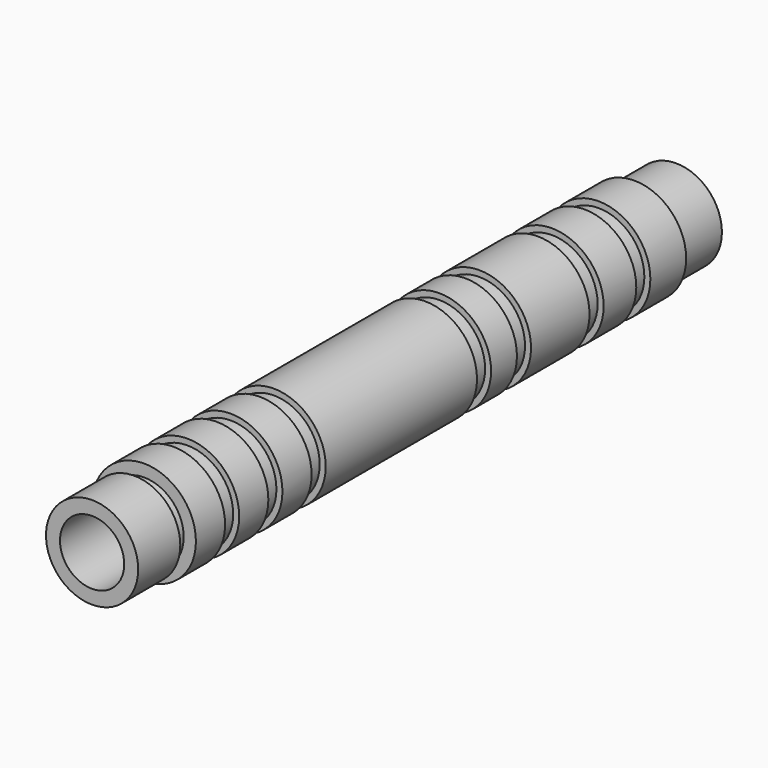
from build123d import *

# Parameters (mm, degrees)
F0_R         = 6.35
F1_DEPTH     = 46.9138
F2_R         = 3.048
F3_DEPTH     = 71.12
F4_R         = 3.937
F5_DEPTH     = 12.3698
F6_R         = 6.35
F6_R_2       = 5.6515
F7_DEPTH     = 6.4516
F8_R         = 6.35
F8_R_2       = 4.8514
F9_DEPTH     = 1.524
F10_S5_R     = 3.937
F10_T6_DEPTH = 7
F12_R        = 6.35
F12_R_2      = 5.6134
F13_DEPTH    = 2.159
F15_R        = 6.35
F15_R_2      = 5.6134
F16_DEPTH    = 2.159
F18_R        = 6.35
F18_R_2      = 5.6134
F19_DEPTH    = 2.159
F21_R        = 6.35
F21_R_2      = 5.6134
F22_DEPTH    = 2.159
F24_R        = 6.35
F24_R_2      = 5.6134
F25_DEPTH    = 2.159
F27_R        = 6.35
F27_R_2      = 5.6134
F28_DEPTH    = 2.159
F30_R        = 6.35
F30_R_2      = 5.6134
F31_DEPTH    = 2.159
F33_R        = 6.35
F33_R_2      = 5.6134
F34_DEPTH    = 10.7198
F35_SIZE2    = 5.6134
F35_SIZE     = 4.318


# Not quite as in the source:
# - a fillet or chamfer that OpenCascade refuses, or shapes differently, is made with other operations: its cross-section is extruded or revolved along the edge and cut away or added


with BuildPart() as f1:
    # F0 (on Front) → F1 (new body, symmetric)
    with BuildSketch(Plane.XZ):
        Circle(F0_R)
    extrude(amount=F1_DEPTH, both=True)

    # F2 (on face) → F3 (cut)
    with BuildSketch(Plane.XZ.offset(46.9138)):
        Circle(F2_R)
    extrude(amount=-F3_DEPTH, mode=Mode.SUBTRACT)

    # F4 (on face) → F5 (cut)
    with BuildSketch(Plane.XZ.offset(46.9138)):
        Circle(F4_R)
    extrude(amount=-F5_DEPTH, mode=Mode.SUBTRACT)

    # F6 (on face) → F7 (cut)
    with BuildSketch(Plane.XZ.offset(46.9138)):
        Circle(F6_R)
        Circle(F6_R_2, mode=Mode.SUBTRACT)
    extrude(amount=-F7_DEPTH, mode=Mode.SUBTRACT)

    # F8 (on face) → F9 (cut)
    with BuildSketch(Plane.XZ.offset(40.4622)):
        Circle(F8_R)
        Circle(F8_R_2, mode=Mode.SUBTRACT)
    extrude(amount=-F9_DEPTH, mode=Mode.SUBTRACT)

    # F10: chamfer of 1.016 on 1 edges, made by hand


with BuildPart() as f10_tool2:
    # F10_s3 → F10_t4 (revolve)
    with BuildSketch(Plane.XY):
        Polygon((4.064, -34.544), (3.048, -33.528), (3.048, -34.544), align=None)
    revolve(axis=Axis((0, -34.544, 0), (0, -1, 0)))

    # F10_s5 → F10_t6 (intersect, symmetric)
    with BuildSketch(Plane.XZ.offset(34)):
        Circle(F10_S5_R)
    extrude(amount=F10_T6_DEPTH, both=True, mode=Mode.INTERSECT)


with BuildPart() as f1_1:
    add(f1.part)

    # F10_t1: cut F10_tool2
    add(f10_tool2.part, mode=Mode.SUBTRACT)

    # F12 (on offset) → F13 (cut)
    with BuildSketch(Plane.XZ.offset(34.4678)):
        Circle(F12_R)
        Circle(F12_R_2, mode=Mode.SUBTRACT)
    extrude(amount=-F13_DEPTH, mode=Mode.SUBTRACT)

    # F15 (on offset) → F16 (cut)
    with BuildSketch(Plane.XZ.offset(27.8384)):
        Circle(F15_R)
        Circle(F15_R_2, mode=Mode.SUBTRACT)
    extrude(amount=-F16_DEPTH, mode=Mode.SUBTRACT)

    # F18 (on offset) → F19 (cut)
    with BuildSketch(Plane.XZ.offset(21.209)):
        Circle(F18_R)
        Circle(F18_R_2, mode=Mode.SUBTRACT)
    extrude(amount=-F19_DEPTH, mode=Mode.SUBTRACT)

    # F21 (on offset) → F22 (cut)
    with BuildSketch(Plane.XZ.offset(-4.1402)):
        Circle(F21_R)
        Circle(F21_R_2, mode=Mode.SUBTRACT)
    extrude(amount=-F22_DEPTH, mode=Mode.SUBTRACT)

    # F24 (on offset) → F25 (cut)
    with BuildSketch(Plane.XZ.offset(-10.2616)):
        Circle(F24_R)
        Circle(F24_R_2, mode=Mode.SUBTRACT)
    extrude(amount=-F25_DEPTH, mode=Mode.SUBTRACT)

    # F27 (on offset) → F28 (cut)
    with BuildSketch(Plane.XZ.offset(-21.3868)):
        Circle(F27_R)
        Circle(F27_R_2, mode=Mode.SUBTRACT)
    extrude(amount=-F28_DEPTH, mode=Mode.SUBTRACT)

    # F30 (on offset) → F31 (cut)
    with BuildSketch(Plane.XZ.offset(-28.5496)):
        Circle(F30_R)
        Circle(F30_R_2, mode=Mode.SUBTRACT)
    extrude(amount=-F31_DEPTH, mode=Mode.SUBTRACT)

    # F33 (on offset) → F34 (cut, through all)
    with BuildSketch(Plane.XZ.offset(-36.195)):
        Circle(F33_R)
        Circle(F33_R_2, mode=Mode.SUBTRACT)
    extrude(amount=-F34_DEPTH, mode=Mode.SUBTRACT)

    # F35
    f35_edges = [f1_1.edges().sort_by_distance(p)[0] for p in [
        (-5.6134, 46.9138, 0),
    ]]
    chamfer(f35_edges, length=F35_SIZE, length2=F35_SIZE2)


solid = f1_1.part
